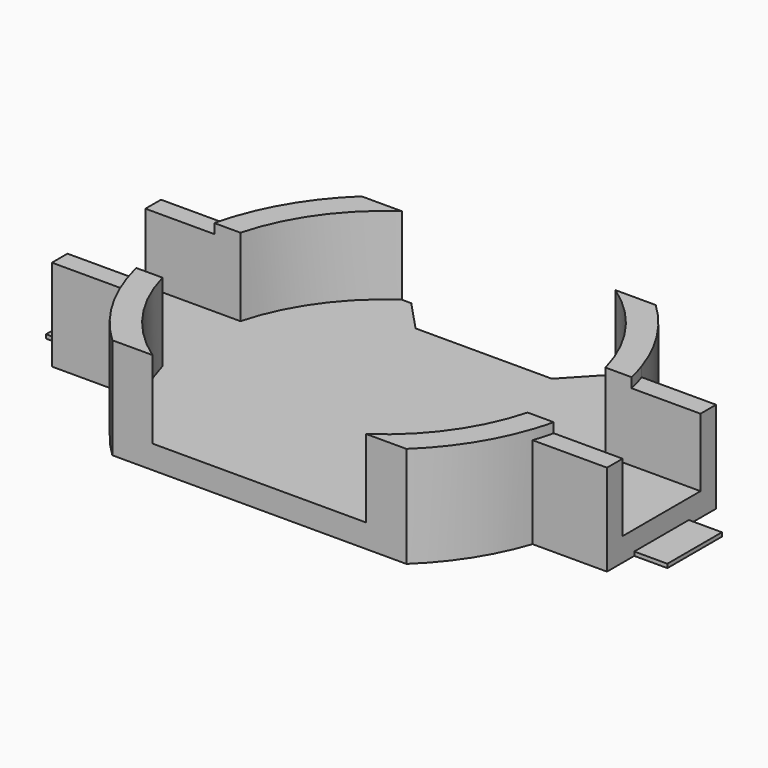
from build123d import *

# Parameters (mm, degrees)
F1_DEPTH = 1.2
F2_DEPTH = 4
F3_DEPTH = 3.5
F4_W     = 1.7
F4_H     = 3.5
F5_DEPTH = 0.2


# Not quite as in the source:
# - a feature names something its author has since deleted; it is built from what else it names


with BuildPart() as f1:
    # F0 (on Top) → F1 (new body)
    with BuildSketch(Plane.XY):
        with BuildLine():
            ThreePointArc((-10.7121426428, 2.5), (-10.5820537772, 3.0033544341), (-10.4283268073, 3.5))
            Line((-10.4283268073, 3.5), (-14.25, 3.5))
            Line((-14.25, 3.5), (-14.25, 2.5))
            Line((-14.25, 2.5), (-10.7121426428, 2.5))
        make_face()
        with BuildLine():
            ThreePointArc((-10.4283268073, -3.5), (-10.5820537772, -3.0033544341), (-10.7121426428, -2.5))
            Line((-10.7121426428, -2.5), (-14.25, -2.5))
            Line((-14.25, -2.5), (-14.25, -3.5))
            Line((-14.25, -3.5), (-10.4283268073, -3.5))
        make_face()
        with BuildLine():
            Line((-9.3722996111, -2.5), (-10.7121426428, -2.5))
            ThreePointArc((-10.7121426428, -2.5), (-10.5820537772, -3.0033544341), (-10.4283268073, -3.5))
            Line((-10.4283268073, -3.5), (-9.0465463023, -3.5))
            ThreePointArc((-9.0465463023, -3.5), (-9.2229860238, -3.004418214), (-9.3722996111, -2.5))
        make_face()
        with BuildLine():
            Line((-9.0465463023, 3.5), (-10.4283268073, 3.5))
            ThreePointArc((-10.4283268073, 3.5), (-10.5820537772, 3.0033544341), (-10.7121426428, 2.5))
            Line((-10.7121426428, 2.5), (-9.3722996111, 2.5))
            ThreePointArc((-9.3722996111, 2.5), (-9.2229860238, 3.004418214), (-9.0465463023, 3.5))
        make_face()
        with BuildLine():
            Line((-9.3722996111, 2.5), (-10.7121426428, 2.5))
            ThreePointArc((-10.7121426428, 2.5), (-11, 0), (-10.7121426428, -2.5))
            Line((-10.7121426428, -2.5), (-9.3722996111, -2.5))
            ThreePointArc((-9.3722996111, -2.5), (-9.7, 0), (-9.3722996111, 2.5))
        make_face()
        with BuildLine():
            ThreePointArc((9.0465463023, 3.5), (7.606386924, 6.0193752136), (5.4854352608, 8))
            Line((5.4854352608, 8), (5, 8))
            Line((5, 8), (3.5, 6.4))
            Line((3.5, 6.4), (-3.5, 6.4))
            Line((-3.5, 6.4), (-5, 8))
            Line((-5, 8), (-5.4854352608, 8))
            ThreePointArc((-5.4854352608, 8), (-7.606386924, 6.0193752136), (-9.0465463023, 3.5))
            Line((-9.0465463023, 3.5), (9.0465463023, 3.5))
        make_face()
        with BuildLine():
            ThreePointArc((9.3722996111, 2.5), (9.2229860238, 3.004418214), (9.0465463023, 3.5))
            Line((9.0465463023, 3.5), (-9.0465463023, 3.5))
            ThreePointArc((-9.0465463023, 3.5), (-9.2229860238, 3.004418214), (-9.3722996111, 2.5))
            ThreePointArc((-9.3722996111, 2.5), (-9.7, 0), (-9.3722996111, -2.5))
            ThreePointArc((-9.3722996111, -2.5), (-9.2229860238, -3.004418214), (-9.0465463023, -3.5))
            Line((-9.0465463023, -3.5), (9.0465463023, -3.5))
            ThreePointArc((9.0465463023, -3.5), (9.2229860238, -3.004418214), (9.3722996111, -2.5))
            ThreePointArc((9.3722996111, -2.5), (9.6177259845, -1.2606930182), (9.7, 0))
            ThreePointArc((9.7, 0), (9.6177259845, 1.2606930182), (9.3722996111, 2.5))
        make_face()
        with BuildLine():
            Line((-5.4854352608, 8), (-7.5498344353, 8))
            ThreePointArc((-7.5498344353, 8), (-9.2663946827, 5.9273880912), (-10.4283268073, 3.5))
            Line((-10.4283268073, 3.5), (-9.0465463023, 3.5))
            ThreePointArc((-9.0465463023, 3.5), (-7.606386924, 6.0193752136), (-5.4854352608, 8))
        make_face()
        with BuildLine():
            ThreePointArc((10.4283268073, 3.5), (9.2663946827, 5.9273880912), (7.5498344353, 8))
            Line((7.5498344353, 8), (5.4854352608, 8))
            ThreePointArc((5.4854352608, 8), (7.606386924, 6.0193752136), (9.0465463023, 3.5))
            Line((9.0465463023, 3.5), (10.4283268073, 3.5))
        make_face()
        with BuildLine():
            Line((14.25, 3.5), (10.4283268073, 3.5))
            ThreePointArc((10.4283268073, 3.5), (10.5820537772, 3.0033544341), (10.7121426428, 2.5))
            Line((10.7121426428, 2.5), (14.25, 2.5))
            Line((14.25, 2.5), (14.25, 3.5))
        make_face()
        with BuildLine():
            Line((14.25, -2.5), (10.7121426428, -2.5))
            ThreePointArc((10.7121426428, -2.5), (10.5820537772, -3.0033544341), (10.4283268073, -3.5))
            Line((10.4283268073, -3.5), (14.25, -3.5))
            Line((14.25, -3.5), (14.25, -2.5))
        make_face()
        with BuildLine():
            ThreePointArc((10.4283268073, -3.5), (10.5820537772, -3.0033544341), (10.7121426428, -2.5))
            Line((10.7121426428, -2.5), (9.3722996111, -2.5))
            ThreePointArc((9.3722996111, -2.5), (9.2229860238, -3.004418214), (9.0465463023, -3.5))
            Line((9.0465463023, -3.5), (10.4283268073, -3.5))
        make_face()
        with BuildLine():
            ThreePointArc((11, 0), (10.9277987049, 1.258258902), (10.7121426428, 2.5))
            Line((10.7121426428, 2.5), (9.3722996111, 2.5))
            ThreePointArc((9.3722996111, 2.5), (9.6177259845, 1.2606930182), (9.7, 0))
            ThreePointArc((9.7, 0), (9.6177259845, -1.2606930182), (9.3722996111, -2.5))
            Line((9.3722996111, -2.5), (10.7121426428, -2.5))
            ThreePointArc((10.7121426428, -2.5), (10.9277987049, -1.258258902), (11, 0))
        make_face()
        with BuildLine():
            ThreePointArc((10.7121426428, 2.5), (10.5820537772, 3.0033544341), (10.4283268073, 3.5))
            Line((10.4283268073, 3.5), (9.0465463023, 3.5))
            ThreePointArc((9.0465463023, 3.5), (9.2229860238, 3.004418214), (9.3722996111, 2.5))
            Line((9.3722996111, 2.5), (10.7121426428, 2.5))
        make_face()
        with BuildLine():
            ThreePointArc((7.5498344353, -8), (9.2663946827, -5.9273880912), (10.4283268073, -3.5))
            Line((10.4283268073, -3.5), (9.0465463023, -3.5))
            ThreePointArc((9.0465463023, -3.5), (7.606386924, -6.0193752136), (5.4854352608, -8))
            Line((5.4854352608, -8), (7.5498344353, -8))
        make_face()
        with BuildLine():
            Line((9.0465463023, -3.5), (-9.0465463023, -3.5))
            ThreePointArc((-9.0465463023, -3.5), (-7.606386924, -6.0193752136), (-5.4854352608, -8))
            Line((-5.4854352608, -8), (5.4854352608, -8))
            ThreePointArc((5.4854352608, -8), (7.606386924, -6.0193752136), (9.0465463023, -3.5))
        make_face()
        with BuildLine():
            Line((-9.0465463023, -3.5), (-10.4283268073, -3.5))
            ThreePointArc((-10.4283268073, -3.5), (-9.2663946827, -5.9273880912), (-7.5498344353, -8))
            Line((-7.5498344353, -8), (-5.4854352608, -8))
            ThreePointArc((-5.4854352608, -8), (-7.606386924, -6.0193752136), (-9.0465463023, -3.5))
        make_face()
        with BuildLine():
            ThreePointArc((-10.7121426428, -2.5), (-11, 0), (-10.7121426428, 2.5))
            Line((-10.7121426428, 2.5), (-14.25, 2.5))
            Line((-14.25, 2.5), (-14.25, -2.5))
            Line((-14.25, -2.5), (-10.7121426428, -2.5))
        make_face()
        with BuildLine():
            Line((14.25, 2.5), (10.7121426428, 2.5))
            ThreePointArc((10.7121426428, 2.5), (10.9277987049, 1.258258902), (11, 0))
            ThreePointArc((11, 0), (10.9277987049, -1.258258902), (10.7121426428, -2.5))
            Line((10.7121426428, -2.5), (14.25, -2.5))
            Line((14.25, -2.5), (14.25, 2.5))
        make_face()
    extrude(amount=-F1_DEPTH)

    # F0 (on Top) → F2 (join)
    with BuildSketch(Plane.XY):
        with BuildLine():
            Line((-5.4854352608, 8), (-7.5498344353, 8))
            ThreePointArc((-7.5498344353, 8), (-9.2663946827, 5.9273880912), (-10.4283268073, 3.5))
            Line((-10.4283268073, 3.5), (-9.0465463023, 3.5))
            ThreePointArc((-9.0465463023, 3.5), (-7.606386924, 6.0193752136), (-5.4854352608, 8))
        make_face()
        with BuildLine():
            Line((-9.0465463023, 3.5), (-10.4283268073, 3.5))
            ThreePointArc((-10.4283268073, 3.5), (-10.5820537772, 3.0033544341), (-10.7121426428, 2.5))
            Line((-10.7121426428, 2.5), (-9.3722996111, 2.5))
            ThreePointArc((-9.3722996111, 2.5), (-9.2229860238, 3.004418214), (-9.0465463023, 3.5))
        make_face()
        with BuildLine():
            Line((-9.3722996111, -2.5), (-10.7121426428, -2.5))
            ThreePointArc((-10.7121426428, -2.5), (-10.5820537772, -3.0033544341), (-10.4283268073, -3.5))
            Line((-10.4283268073, -3.5), (-9.0465463023, -3.5))
            ThreePointArc((-9.0465463023, -3.5), (-9.2229860238, -3.004418214), (-9.3722996111, -2.5))
        make_face()
        with BuildLine():
            Line((-9.0465463023, -3.5), (-10.4283268073, -3.5))
            ThreePointArc((-10.4283268073, -3.5), (-9.2663946827, -5.9273880912), (-7.5498344353, -8))
            Line((-7.5498344353, -8), (-5.4854352608, -8))
            ThreePointArc((-5.4854352608, -8), (-7.606386924, -6.0193752136), (-9.0465463023, -3.5))
        make_face()
        with BuildLine():
            ThreePointArc((7.5498344353, -8), (9.2663946827, -5.9273880912), (10.4283268073, -3.5))
            Line((10.4283268073, -3.5), (9.0465463023, -3.5))
            ThreePointArc((9.0465463023, -3.5), (7.606386924, -6.0193752136), (5.4854352608, -8))
            Line((5.4854352608, -8), (7.5498344353, -8))
        make_face()
        with BuildLine():
            ThreePointArc((10.4283268073, -3.5), (10.5820537772, -3.0033544341), (10.7121426428, -2.5))
            Line((10.7121426428, -2.5), (9.3722996111, -2.5))
            ThreePointArc((9.3722996111, -2.5), (9.2229860238, -3.004418214), (9.0465463023, -3.5))
            Line((9.0465463023, -3.5), (10.4283268073, -3.5))
        make_face()
        with BuildLine():
            ThreePointArc((10.4283268073, 3.5), (9.2663946827, 5.9273880912), (7.5498344353, 8))
            Line((7.5498344353, 8), (5.4854352608, 8))
            ThreePointArc((5.4854352608, 8), (7.606386924, 6.0193752136), (9.0465463023, 3.5))
            Line((9.0465463023, 3.5), (10.4283268073, 3.5))
        make_face()
        with BuildLine():
            ThreePointArc((10.7121426428, 2.5), (10.5820537772, 3.0033544341), (10.4283268073, 3.5))
            Line((10.4283268073, 3.5), (9.0465463023, 3.5))
            ThreePointArc((9.0465463023, 3.5), (9.2229860238, 3.004418214), (9.3722996111, 2.5))
            Line((9.3722996111, 2.5), (10.7121426428, 2.5))
        make_face()
    extrude(amount=F2_DEPTH)

    # F0 (on Top) → F3 (join)
    with BuildSketch(Plane.XY):
        with BuildLine():
            ThreePointArc((-10.7121426428, 2.5), (-10.5820537772, 3.0033544341), (-10.4283268073, 3.5))
            Line((-10.4283268073, 3.5), (-14.25, 3.5))
            Line((-14.25, 3.5), (-14.25, 2.5))
            Line((-14.25, 2.5), (-10.7121426428, 2.5))
        make_face()
        with BuildLine():
            ThreePointArc((-10.4283268073, -3.5), (-10.5820537772, -3.0033544341), (-10.7121426428, -2.5))
            Line((-10.7121426428, -2.5), (-14.25, -2.5))
            Line((-14.25, -2.5), (-14.25, -3.5))
            Line((-14.25, -3.5), (-10.4283268073, -3.5))
        make_face()
        with BuildLine():
            Line((14.25, -2.5), (10.7121426428, -2.5))
            ThreePointArc((10.7121426428, -2.5), (10.5820537772, -3.0033544341), (10.4283268073, -3.5))
            Line((10.4283268073, -3.5), (14.25, -3.5))
            Line((14.25, -3.5), (14.25, -2.5))
        make_face()
        with BuildLine():
            Line((14.25, 3.5), (10.4283268073, 3.5))
            ThreePointArc((10.4283268073, 3.5), (10.5820537772, 3.0033544341), (10.7121426428, 2.5))
            Line((10.7121426428, 2.5), (14.25, 2.5))
            Line((14.25, 2.5), (14.25, 3.5))
        make_face()
    extrude(amount=F3_DEPTH)

    # F4 (on face) → F5 (join)
    with BuildSketch(Plane(origin=(0, 0, -1.2), x_dir=(1, 0, 0), z_dir=(0, 0, -1))):
        with Locations((-15.1, 0)):
            Rectangle(F4_W, F4_H)
        with Locations((15.1, 0)):
            Rectangle(F4_W, F4_H)
    extrude(amount=-F5_DEPTH)


solid = f1.part
